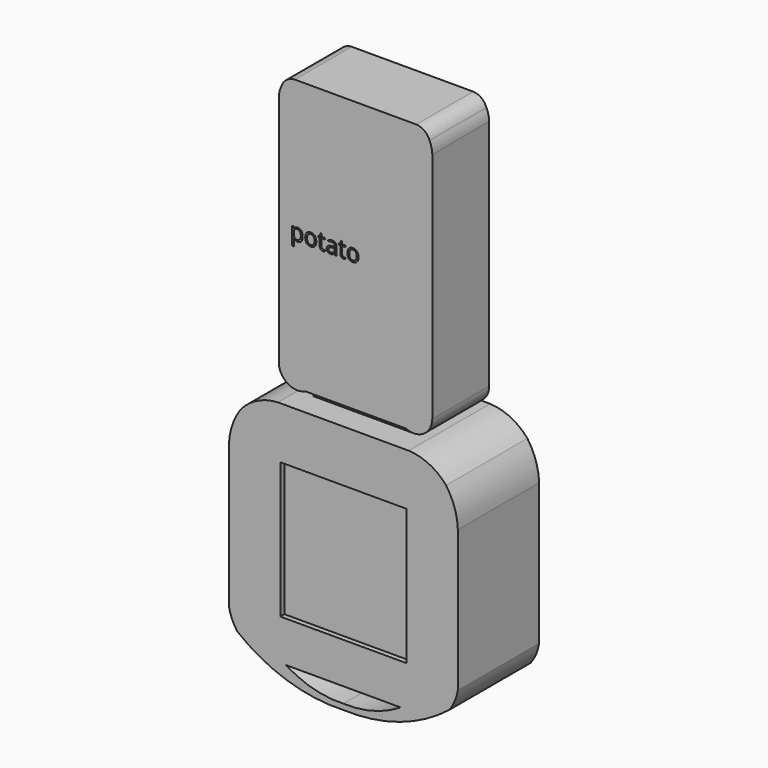
from build123d import *

# Parameters (mm, degrees)
F1_DEPTH      = 7
F1_DEPTH_BACK = 7
F0_W          = 19.7578053921
F0_H          = 1.6641734354
F2_DEPTH      = 5
F2_DEPTH_BACK = 5
F3_DEPTH      = 10
F3_DEPTH_BACK = 10
F0_W_2        = 24.8230153336
F0_H_2        = 26.7400959404
F0_R          = 11.1738098935
F4_DEPTH      = 9
F4_DEPTH_BACK = 8
F0_TEXT_SIZE  = 4.4513079855
F5_DEPTH      = 6
F5_DEPTH_BACK = 6
F6_DEPTH      = 10
F6_DEPTH_BACK = 8
F7_DEPTH      = 9
F7_DEPTH_BACK = 10


# Not quite as in the source:
# - Text() gives the source's letters only with a copy of the font that has no kerning and outlines rounded to 1/6400 em; it was checked with that copy


with BuildPart() as f1:
    # F0 (on Front) → F1 (new body, two sides)
    with BuildSketch(Plane.XZ) as f1_sk:
        with BuildLine():
            ThreePointArc((-0.3371863552, 48.0720782434), (-1.3488067521, 49.4383829581), (-2.9534097244, 50))
            Line((-2.9534097244, 50), (-3.174751997, 50))
            Line((-3.174751997, 50), (-14.9015085772, 50))
            Line((-14.9015085772, 50), (-26.6282651573, 50))
            Line((-26.6282651573, 50), (-26.8496074299, 50))
            ThreePointArc((-26.8496074299, 50), (-28.4542104022, 49.4383829581), (-29.4658307991, 48.0720782434))
            ThreePointArc((-29.4658307991, 48.0720782434), (-29.8531970792, 46.9903534646), (-30, 45.8507789675))
            Line((-30, 45.8507789675), (-30, 45.6348136067))
            Line((-30, 45.6348136067), (-30, 0))
            ThreePointArc((-30, 0), (-28.3036916744, -3.0972506092), (-24.7804112732, -3.3358265646))
            Line((-24.7804112732, -3.3358265646), (-5.0226058811, -3.3358265646))
            ThreePointArc((-5.0226058811, -3.3358265646), (-1.4993254799, -3.0972506092), (0.1969828457, 0))
            Line((0.1969828457, 0), (0.1969828457, 45.6348136067))
            Line((0.1969828457, 45.6348136067), (0.1969828457, 45.8507789675))
            ThreePointArc((0.1969828457, 45.8507789675), (0.0501799248, 46.9903534646), (-0.3371863552, 48.0720782434))
        make_face()
        with BuildLine():
            add(Edge.make_bspline(
                [(-25.5638879543, 22.3995790325), (-25.8257500569, 22.0744248945), (-26.2910508447, 22.0744248945)],
                knots=[0, 0, 0, 1, 1, 1], degree=2))
            add(Edge.make_bspline(
                [(-26.2910508447, 22.0744248945), (-26.5240489971, 22.0744248945), (-26.7163594124, 22.1603212283)],
                knots=[0, 0, 0, 1, 1, 1], degree=2))
            add(Edge.make_bspline(
                [(-26.7163594124, 22.1603212283), (-26.9086698277, 22.2462175621), (-27.0387314829, 22.4249653984)],
                knots=[0, 0, 0, 1, 1, 1], degree=2))
            Line((-27.0387314829, 22.4249653984), (-27.0651611241, 22.4249653984))
            add(Edge.make_bspline(
                [(-27.0651611241, 22.4249653984), (-27.0387314829, 22.2163103366), (-27.0387314829, 22.0292162978)],
                knots=[0, 0, 0, 1, 1, 1], degree=2))
            Line((-27.0387314829, 22.0292162978), (-27.0387314829, 21.0485375072))
            Line((-27.0387314829, 21.0485375072), (-27.3997047399, 21.0485375072))
            Line((-27.3997047399, 21.0485375072), (-27.3997047399, 24.5003877466))
            Line((-27.3997047399, 24.5003877466), (-27.1061966196, 24.5003877466))
            Line((-27.1061966196, 24.5003877466), (-27.0561194047, 24.1741903333))
            Line((-27.0561194047, 24.1741903333), (-27.0387314829, 24.1741903333))
            add(Edge.make_bspline(
                [(-27.0387314829, 24.1741903333), (-26.8996281084, 24.3703260914), (-26.7149683787, 24.4572657005)],
                knots=[0, 0, 0, 1, 1, 1], degree=2))
            add(Edge.make_bspline(
                [(-26.7149683787, 24.4572657005), (-26.5303086489, 24.5442053096), (-26.2910508447, 24.5442053096)],
                knots=[0, 0, 0, 1, 1, 1], degree=2))
            add(Edge.make_bspline(
                [(-26.2910508447, 24.5442053096), (-25.8174038544, 24.5442053096), (-25.559714853, 24.2200944469)],
                knots=[0, 0, 0, 1, 1, 1], degree=2))
            add(Edge.make_bspline(
                [(-25.559714853, 24.2200944469), (-25.3020258517, 23.8959835842), (-25.3020258517, 23.3117494111)],
                knots=[0, 0, 0, 1, 1, 1], degree=2))
            add(Edge.make_bspline(
                [(-25.3020258517, 23.3117494111), (-25.3020258517, 22.7247331705), (-25.5638879543, 22.3995790325)],
                knots=[0, 0, 0, 1, 1, 1], degree=2))
        make_face(mode=Mode.SUBTRACT)
        with BuildLine():
            add(Edge.make_bspline(
                [(-22.9104910848, 24.211400486), (-22.6159396892, 23.8785956624), (-22.6159396892, 23.3117494111)],
                knots=[0, 0, 0, 1, 1, 1], degree=2))
            add(Edge.make_bspline(
                [(-22.6159396892, 23.3117494111), (-22.6159396892, 22.7289062718), (-22.909100051, 22.4016655831)],
                knots=[0, 0, 0, 1, 1, 1], degree=2))
            add(Edge.make_bspline(
                [(-22.909100051, 22.4016655831), (-23.2022604129, 22.0744248945), (-23.7197249662, 22.0744248945)],
                knots=[0, 0, 0, 1, 1, 1], degree=2))
            add(Edge.make_bspline(
                [(-23.7197249662, 22.0744248945), (-24.0396627277, 22.0744248945), (-24.2872667344, 22.224656539)],
                knots=[0, 0, 0, 1, 1, 1], degree=2))
            add(Edge.make_bspline(
                [(-24.2872667344, 22.224656539), (-24.5348707411, 22.3748881835), (-24.6698010144, 22.6551814833)],
                knots=[0, 0, 0, 1, 1, 1], degree=2))
            add(Edge.make_bspline(
                [(-24.6698010144, 22.6551814833), (-24.8047312877, 22.935474783), (-24.8047312877, 23.3117494111)],
                knots=[0, 0, 0, 1, 1, 1], degree=2))
            add(Edge.make_bspline(
                [(-24.8047312877, 23.3117494111), (-24.8047312877, 23.8938970336), (-24.513309718, 24.2190511716)],
                knots=[0, 0, 0, 1, 1, 1], degree=2))
            add(Edge.make_bspline(
                [(-24.513309718, 24.2190511716), (-24.2218881483, 24.5442053096), (-23.704423595, 24.5442053096)],
                knots=[0, 0, 0, 1, 1, 1], degree=2))
            add(Edge.make_bspline(
                [(-23.704423595, 24.5442053096), (-23.2050424804, 24.5442053096), (-22.9104910848, 24.211400486)],
                knots=[0, 0, 0, 1, 1, 1], degree=2))
        make_face(mode=Mode.SUBTRACT)
        with BuildLine():
            add(Edge.make_bspline(
                [(-21.4940709735, 22.4879096754), (-21.3918299932, 22.3728016329), (-21.2137776737, 22.3728016329)],
                knots=[0, 0, 0, 1, 1, 1], degree=2))
            add(Edge.make_bspline(
                [(-21.2137776737, 22.3728016329), (-21.1177963453, 22.3728016329), (-21.0287701856, 22.3867119704)],
                knots=[0, 0, 0, 1, 1, 1], degree=2))
            add(Edge.make_bspline(
                [(-21.0287701856, 22.3867119704), (-20.9397440259, 22.4006223078), (-20.8875802604, 22.415923679)],
                knots=[0, 0, 0, 1, 1, 1], degree=2))
            Line((-20.8875802604, 22.415923679), (-20.8875802604, 22.1398034806))
            add(Edge.make_bspline(
                [(-20.8875802604, 22.1398034806), (-20.9460036777, 22.1119828057), (-21.0600684449, 22.0932038501)],
                knots=[0, 0, 0, 1, 1, 1], degree=2))
            add(Edge.make_bspline(
                [(-21.0600684449, 22.0932038501), (-21.174133212, 22.0744248945), (-21.2659414392, 22.0744248945)],
                knots=[0, 0, 0, 1, 1, 1], degree=2))
            add(Edge.make_bspline(
                [(-21.2659414392, 22.0744248945), (-21.9565896938, 22.0744248945), (-21.9565896938, 22.8026310603)],
                knots=[0, 0, 0, 1, 1, 1], degree=2))
            Line((-21.9565896938, 22.8026310603), (-21.9565896938, 24.2200944469))
            Line((-21.9565896938, 24.2200944469), (-22.2980884783, 24.2200944469))
            Line((-22.2980884783, 24.2200944469), (-22.2980884783, 24.3939736651))
            Line((-22.2980884783, 24.3939736651), (-21.9565896938, 24.5442053096))
            Line((-21.9565896938, 24.5442053096), (-21.8049670156, 25.0526281436))
            Line((-21.8049670156, 25.0526281436), (-21.5963119537, 25.0526281436))
            Line((-21.5963119537, 25.0526281436), (-21.5963119537, 24.5003877466))
            Line((-21.5963119537, 24.5003877466), (-20.9049681822, 24.5003877466))
            Line((-20.9049681822, 24.5003877466), (-20.9049681822, 24.2200944469))
            Line((-20.9049681822, 24.2200944469), (-21.5963119537, 24.2200944469))
            Line((-21.5963119537, 24.2200944469), (-21.5963119537, 22.8179324315))
            add(Edge.make_bspline(
                [(-21.5963119537, 22.8179324315), (-21.5963119537, 22.6030177178), (-21.4940709735, 22.4879096754)],
                knots=[0, 0, 0, 1, 1, 1], degree=2))
        make_face(mode=Mode.SUBTRACT)
        with BuildLine():
            Line((-18.6793141895, 22.1182424575), (-18.9470881855, 22.1182424575))
            Line((-18.9470881855, 22.1182424575), (-19.0187264234, 22.4576546914))
            Line((-19.0187264234, 22.4576546914), (-19.0361143452, 22.4576546914))
            add(Edge.make_bspline(
                [(-19.0361143452, 22.4576546914), (-19.2141666646, 22.2336982584), (-19.3911757087, 22.1540615765)],
                knots=[0, 0, 0, 1, 1, 1], degree=2))
            add(Edge.make_bspline(
                [(-19.3911757087, 22.1540615765), (-19.5681847528, 22.0744248945), (-19.8338721982, 22.0744248945)],
                knots=[0, 0, 0, 1, 1, 1], degree=2))
            add(Edge.make_bspline(
                [(-19.8338721982, 22.0744248945), (-20.1878902865, 22.0744248945), (-20.3888946627, 22.2573458321)],
                knots=[0, 0, 0, 1, 1, 1], degree=2))
            add(Edge.make_bspline(
                [(-20.3888946627, 22.2573458321), (-20.5898990389, 22.4402667696), (-20.5898990389, 22.776896936)],
                knots=[0, 0, 0, 1, 1, 1], degree=2))
            add(Edge.make_bspline(
                [(-20.5898990389, 22.776896936), (-20.5898990389, 23.498147933), (-19.436036547, 23.5329237767)],
                knots=[0, 0, 0, 1, 1, 1], degree=2))
            Line((-19.436036547, 23.5329237767), (-19.031941244, 23.5461385972))
            Line((-19.031941244, 23.5461385972), (-19.031941244, 23.6942836911))
            add(Edge.make_bspline(
                [(-19.031941244, 23.6942836911), (-19.031941244, 23.9745769908), (-19.1522656629, 24.1081162304)],
                knots=[0, 0, 0, 1, 1, 1], degree=2))
            add(Edge.make_bspline(
                [(-19.1522656629, 24.1081162304), (-19.2725900819, 24.24165547), (-19.5382775273, 24.24165547)],
                knots=[0, 0, 0, 1, 1, 1], degree=2))
            add(Edge.make_bspline(
                [(-19.5382775273, 24.24165547), (-19.8359587488, 24.24165547), (-20.2115378601, 24.0594300493)],
                knots=[0, 0, 0, 1, 1, 1], degree=2))
            Line((-20.2115378601, 24.0594300493), (-20.3228205598, 24.3355502478))
            add(Edge.make_bspline(
                [(-20.3228205598, 24.3355502478), (-20.146854791, 24.4308360594), (-19.9371564538, 24.4850863754)],
                knots=[0, 0, 0, 1, 1, 1], degree=2))
            add(Edge.make_bspline(
                [(-19.9371564538, 24.4850863754), (-19.7274581167, 24.5393366915), (-19.5160209874, 24.5393366915)],
                knots=[0, 0, 0, 1, 1, 1], degree=2))
            add(Edge.make_bspline(
                [(-19.5160209874, 24.5393366915), (-19.0903646613, 24.5393366915), (-18.8848394254, 24.3505038606)],
                knots=[0, 0, 0, 1, 1, 1], degree=2))
            add(Edge.make_bspline(
                [(-18.8848394254, 24.3505038606), (-18.6793141895, 24.1616710296), (-18.6793141895, 23.744360906)],
                knots=[0, 0, 0, 1, 1, 1], degree=2))
            Line((-18.6793141895, 23.744360906), (-18.6793141895, 22.1182424575))
        make_face(mode=Mode.SUBTRACT)
        with BuildLine():
            add(Edge.make_bspline(
                [(-17.4475538079, 22.4879096754), (-17.3453128276, 22.3728016329), (-17.1672605082, 22.3728016329)],
                knots=[0, 0, 0, 1, 1, 1], degree=2))
            add(Edge.make_bspline(
                [(-17.1672605082, 22.3728016329), (-17.0712791797, 22.3728016329), (-16.98225302, 22.3867119704)],
                knots=[0, 0, 0, 1, 1, 1], degree=2))
            add(Edge.make_bspline(
                [(-16.98225302, 22.3867119704), (-16.8932268603, 22.4006223078), (-16.8410630948, 22.415923679)],
                knots=[0, 0, 0, 1, 1, 1], degree=2))
            Line((-16.8410630948, 22.415923679), (-16.8410630948, 22.1398034806))
            add(Edge.make_bspline(
                [(-16.8410630948, 22.1398034806), (-16.8994865122, 22.1119828057), (-17.0135512793, 22.0932038501)],
                knots=[0, 0, 0, 1, 1, 1], degree=2))
            add(Edge.make_bspline(
                [(-17.0135512793, 22.0932038501), (-17.1276160464, 22.0744248945), (-17.2194242736, 22.0744248945)],
                knots=[0, 0, 0, 1, 1, 1], degree=2))
            add(Edge.make_bspline(
                [(-17.2194242736, 22.0744248945), (-17.9100725282, 22.0744248945), (-17.9100725282, 22.8026310603)],
                knots=[0, 0, 0, 1, 1, 1], degree=2))
            Line((-17.9100725282, 22.8026310603), (-17.9100725282, 24.2200944469))
            Line((-17.9100725282, 24.2200944469), (-18.2515713128, 24.2200944469))
            Line((-18.2515713128, 24.2200944469), (-18.2515713128, 24.3939736651))
            Line((-18.2515713128, 24.3939736651), (-17.9100725282, 24.5442053096))
            Line((-17.9100725282, 24.5442053096), (-17.75844985, 25.0526281436))
            Line((-17.75844985, 25.0526281436), (-17.5497947882, 25.0526281436))
            Line((-17.5497947882, 25.0526281436), (-17.5497947882, 24.5003877466))
            Line((-17.5497947882, 24.5003877466), (-16.8584510167, 24.5003877466))
            Line((-16.8584510167, 24.5003877466), (-16.8584510167, 24.2200944469))
            Line((-16.8584510167, 24.2200944469), (-17.5497947882, 24.2200944469))
            Line((-17.5497947882, 24.2200944469), (-17.5497947882, 22.8179324315))
            add(Edge.make_bspline(
                [(-17.5497947882, 22.8179324315), (-17.5497947882, 22.6030177178), (-17.4475538079, 22.4879096754)],
                knots=[0, 0, 0, 1, 1, 1], degree=2))
        make_face(mode=Mode.SUBTRACT)
        with BuildLine():
            add(Edge.make_bspline(
                [(-14.6039330737, 24.211400486), (-14.3093816781, 23.8785956624), (-14.3093816781, 23.3117494111)],
                knots=[0, 0, 0, 1, 1, 1], degree=2))
            add(Edge.make_bspline(
                [(-14.3093816781, 23.3117494111), (-14.3093816781, 22.7289062718), (-14.6025420399, 22.4016655831)],
                knots=[0, 0, 0, 1, 1, 1], degree=2))
            add(Edge.make_bspline(
                [(-14.6025420399, 22.4016655831), (-14.8957024018, 22.0744248945), (-15.4131669551, 22.0744248945)],
                knots=[0, 0, 0, 1, 1, 1], degree=2))
            add(Edge.make_bspline(
                [(-15.4131669551, 22.0744248945), (-15.7331047166, 22.0744248945), (-15.9807087233, 22.224656539)],
                knots=[0, 0, 0, 1, 1, 1], degree=2))
            add(Edge.make_bspline(
                [(-15.9807087233, 22.224656539), (-16.22831273, 22.3748881835), (-16.3632430033, 22.6551814833)],
                knots=[0, 0, 0, 1, 1, 1], degree=2))
            add(Edge.make_bspline(
                [(-16.3632430033, 22.6551814833), (-16.4981732766, 22.935474783), (-16.4981732766, 23.3117494111)],
                knots=[0, 0, 0, 1, 1, 1], degree=2))
            add(Edge.make_bspline(
                [(-16.4981732766, 23.3117494111), (-16.4981732766, 23.8938970336), (-16.2067517069, 24.2190511716)],
                knots=[0, 0, 0, 1, 1, 1], degree=2))
            add(Edge.make_bspline(
                [(-16.2067517069, 24.2190511716), (-15.9153301372, 24.5442053096), (-15.3978655839, 24.5442053096)],
                knots=[0, 0, 0, 1, 1, 1], degree=2))
            add(Edge.make_bspline(
                [(-15.3978655839, 24.5442053096), (-14.8984844693, 24.5442053096), (-14.6039330737, 24.211400486)],
                knots=[0, 0, 0, 1, 1, 1], degree=2))
        make_face(mode=Mode.SUBTRACT)
    extrude(amount=F1_DEPTH)
    extrude(f1_sk.sketch, amount=-F1_DEPTH_BACK)

    # F0 (on Front) → F2 (join, two sides)
    with BuildSketch(Plane.XZ) as f2_sk:
        with Locations((-14.9015085772, -4.1679132823)):
            Rectangle(F0_W, F0_H)
    extrude(amount=F2_DEPTH)
    extrude(f2_sk.sketch, amount=-F2_DEPTH_BACK)

    # F0 (on Front) → F3 (join, two sides)
    with BuildSketch(Plane.XZ) as f3_sk:
        with BuildLine():
            Line((-4.7804112732, -5), (-5.0226058811, -5))
            Line((-5.0226058811, -5), (-24.7804112732, -5))
            Line((-24.7804112732, -5), (-26.8505178392, -5))
            Line((-26.8505178392, -5), (-27.7755146487, -5))
            ThreePointArc((-27.7755146487, -5), (-31.8249756764, -6.0389542539), (-35.1200683324, -8.6118757345))
            ThreePointArc((-35.1200683324, -8.6118757345), (-36.7849914207, -11.9049706979), (-37.4285317957, -15.5384675143))
            Line((-37.4285317957, -15.5384675143), (-37.4285317957, -43.3827936649))
            ThreePointArc((-37.4285317957, -43.3827936649), (-36.8364830132, -45.4381899261), (-35.7731175765, -47.2941073539))
            ThreePointArc((-35.7731175765, -47.2941073539), (-25.9517344842, -52.5831834244), (-14.9015085772, -54.1084371507))
            ThreePointArc((-14.9015085772, -54.1084371507), (-3.8512826702, -52.5831834244), (5.9701004222, -47.2941073539))
            ThreePointArc((5.9701004222, -47.2941073539), (7.0334658589, -45.4381899261), (7.6255146414, -43.3827936649))
            Line((7.6255146414, -43.3827936649), (7.6255146414, -15.5384675143))
            ThreePointArc((7.6255146414, -15.5384675143), (6.9819742664, -11.9049706979), (5.317051178, -8.6118757345))
            ThreePointArc((5.317051178, -8.6118757345), (2.0219585221, -6.0389542539), (-2.0275025056, -5))
            Line((-2.0275025056, -5), (-2.9524993151, -5))
            Line((-2.9524993151, -5), (-4.7804112732, -5))
        make_face()
        with BuildLine():
            ThreePointArc((-3.6269985139, -50), (-9.0351634562, -52.3629954978), (-14.9015085772, -53.0095174909))
            ThreePointArc((-14.9015085772, -53.0095174909), (-20.7678536981, -52.3629954978), (-26.1760186404, -50))
            Line((-26.1760186404, -50), (-3.6269985139, -50))
        make_face(mode=Mode.SUBTRACT)
        Polygon((-2.4900009104, -41.9538753285), (-27.313016244, -41.9538753285), (-28.6317821592, -41.9538753285), (-28.6317821592, -13.223904185), (-1.1990642376, -13.223904185), (-1.1990642376, -41.9538753285), align=None, mode=Mode.SUBTRACT)
    extrude(amount=F3_DEPTH)
    extrude(f3_sk.sketch, amount=-F3_DEPTH_BACK)

    # F0 (on Front) → F4 (join, two sides)
    with BuildSketch(Plane.XZ) as f4_sk:
        with Locations((-14.9015085772, -28.5838273583)):
            Rectangle(F0_W_2, F0_H_2)
        with Locations((-14.8883853108, -28.2334722579)):
            Circle(F0_R, mode=Mode.SUBTRACT)
    extrude(amount=F4_DEPTH)
    extrude(f4_sk.sketch, amount=-F4_DEPTH_BACK)

    # F0 (on Front) → F6 (join, two sides)
    with BuildSketch(Plane.XZ) as f6_sk:
        Polygon((-27.313016244, -41.9538753285), (-27.313016244, -15.2137793881), (-2.4900009104, -15.2137793881), (-2.4900009104, -41.9538753285), (-1.1990642376, -41.9538753285), (-1.1990642376, -13.223904185), (-28.6317821592, -13.223904185), (-28.6317821592, -41.9538753285), align=None)
    extrude(amount=F6_DEPTH)
    extrude(f6_sk.sketch, amount=-F6_DEPTH_BACK)

    # F0 (on Front) → F7 (join, two sides)
    with BuildSketch(Plane.XZ) as f7_sk:
        with Locations((-14.8883853108, -28.2334722579)):
            Circle(F0_R)
    extrude(amount=F7_DEPTH)
    extrude(f7_sk.sketch, amount=-F7_DEPTH_BACK)


with BuildPart() as f1b:
    # F0 (on Front) → F1, piece 2 (new body, two sides)
    with BuildSketch(Plane.XZ) as f1_2_sk:
        with BuildLine():
            add(Edge.make_bspline(
                [(-24.2500565817, 24.0048319748), (-24.4305432102, 23.7721815809), (-24.4305432102, 23.3117494111)],
                knots=[0, 0, 0, 1, 1, 1], degree=2))
            add(Edge.make_bspline(
                [(-24.4305432102, 23.3117494111), (-24.4305432102, 22.8547948257), (-24.2479700311, 22.61588478)],
                knots=[0, 0, 0, 1, 1, 1], degree=2))
            add(Edge.make_bspline(
                [(-24.2479700311, 22.61588478), (-24.065396852, 22.3769747342), (-23.7113787637, 22.3769747342)],
                knots=[0, 0, 0, 1, 1, 1], degree=2))
            add(Edge.make_bspline(
                [(-23.7113787637, 22.3769747342), (-23.3566651586, 22.3769747342), (-23.1730487042, 22.6148415046)],
                knots=[0, 0, 0, 1, 1, 1], degree=2))
            add(Edge.make_bspline(
                [(-23.1730487042, 22.6148415046), (-22.9894322498, 22.8527082751), (-22.9894322498, 23.3117494111)],
                knots=[0, 0, 0, 1, 1, 1], degree=2))
            add(Edge.make_bspline(
                [(-22.9894322498, 23.3117494111), (-22.9894322498, 23.765921929), (-23.1730487042, 24.0017021489)],
                knots=[0, 0, 0, 1, 1, 1], degree=2))
            add(Edge.make_bspline(
                [(-23.1730487042, 24.0017021489), (-23.3566651586, 24.2374823687), (-23.715551865, 24.2374823687)],
                knots=[0, 0, 0, 1, 1, 1], degree=2))
            add(Edge.make_bspline(
                [(-23.715551865, 24.2374823687), (-24.0695699532, 24.2374823687), (-24.2500565817, 24.0048319748)],
                knots=[0, 0, 0, 1, 1, 1], degree=2))
        make_face()
    extrude(amount=F1_DEPTH)
    extrude(f1_2_sk.sketch, amount=-F1_DEPTH_BACK)


with BuildPart() as f1c:
    # F0 (on Front) → F1, piece 3 (new body, two sides)
    with BuildSketch(Plane.XZ) as f1_3_sk:
        with BuildLine():
            add(Edge.make_bspline(
                [(-25.8511364227, 23.9996155983), (-26.0260589162, 24.2374823687), (-26.3432146102, 24.2374823687)],
                knots=[0, 0, 0, 1, 1, 1], degree=2))
            add(Edge.make_bspline(
                [(-26.3432146102, 24.2374823687), (-26.7083609684, 24.2374823687), (-26.871459675, 24.0354347172)],
                knots=[0, 0, 0, 1, 1, 1], degree=2))
            add(Edge.make_bspline(
                [(-26.871459675, 24.0354347172), (-27.0345583817, 23.8333870657), (-27.0387314829, 23.3917338515)],
                knots=[0, 0, 0, 1, 1, 1], degree=2))
            Line((-27.0387314829, 23.3917338515), (-27.0387314829, 23.3117494111))
            add(Edge.make_bspline(
                [(-27.0387314829, 23.3117494111), (-27.0387314829, 22.809586229), (-26.871459675, 22.5932804816)],
                knots=[0, 0, 0, 1, 1, 1], degree=2))
            add(Edge.make_bspline(
                [(-26.871459675, 22.5932804816), (-26.7041878671, 22.3769747342), (-26.3348684077, 22.3769747342)],
                knots=[0, 0, 0, 1, 1, 1], degree=2))
            add(Edge.make_bspline(
                [(-26.3348684077, 22.3769747342), (-26.0260589162, 22.3769747342), (-25.8511364227, 22.6270130499)],
                knots=[0, 0, 0, 1, 1, 1], degree=2))
            add(Edge.make_bspline(
                [(-25.8511364227, 22.6270130499), (-25.6762139292, 22.8770513657), (-25.6762139292, 23.3159225124)],
                knots=[0, 0, 0, 1, 1, 1], degree=2))
            add(Edge.make_bspline(
                [(-25.6762139292, 23.3159225124), (-25.6762139292, 23.7617488278), (-25.8511364227, 23.9996155983)],
                knots=[0, 0, 0, 1, 1, 1], degree=2))
        make_face()
    extrude(amount=F1_DEPTH)
    extrude(f1_3_sk.sketch, amount=-F1_DEPTH_BACK)


with BuildPart() as f1d:
    # F0 (on Front) → F1, piece 4 (new body, two sides)
    with BuildSketch(Plane.XZ) as f1_4_sk:
        with BuildLine():
            add(Edge.make_bspline(
                [(-20.0932999918, 22.4746948548), (-19.9750621234, 22.3728016329), (-19.7622339603, 22.3728016329)],
                knots=[0, 0, 0, 1, 1, 1], degree=2))
            add(Edge.make_bspline(
                [(-19.7622339603, 22.3728016329), (-19.4249082771, 22.3728016329), (-19.2325978617, 22.5574613626)],
                knots=[0, 0, 0, 1, 1, 1], degree=2))
            add(Edge.make_bspline(
                [(-19.2325978617, 22.5574613626), (-19.0402874464, 22.7421210924), (-19.0402874464, 23.0745781575)],
                knots=[0, 0, 0, 1, 1, 1], degree=2))
            Line((-19.0402874464, 23.0745781575), (-19.0402874464, 23.2894928712))
            Line((-19.0402874464, 23.2894928712), (-19.4012607034, 23.2748870169))
            add(Edge.make_bspline(
                [(-19.4012607034, 23.2748870169), (-19.8317856476, 23.2595856457), (-20.0216617539, 23.1410000189)],
                knots=[0, 0, 0, 1, 1, 1], degree=2))
            add(Edge.make_bspline(
                [(-20.0216617539, 23.1410000189), (-20.2115378601, 23.0224143921), (-20.2115378601, 22.7727238348)],
                knots=[0, 0, 0, 1, 1, 1], degree=2))
            add(Edge.make_bspline(
                [(-20.2115378601, 22.7727238348), (-20.2115378601, 22.5765880766), (-20.0932999918, 22.4746948548)],
                knots=[0, 0, 0, 1, 1, 1], degree=2))
        make_face()
    extrude(amount=F1_DEPTH)
    extrude(f1_4_sk.sketch, amount=-F1_DEPTH_BACK)


with BuildPart() as f1e:
    # F0 (on Front) → F1, piece 5 (new body, two sides)
    with BuildSketch(Plane.XZ) as f1_5_sk:
        with BuildLine():
            add(Edge.make_bspline(
                [(-15.9434985706, 24.0048319748), (-16.1239851991, 23.7721815809), (-16.1239851991, 23.3117494111)],
                knots=[0, 0, 0, 1, 1, 1], degree=2))
            add(Edge.make_bspline(
                [(-16.1239851991, 23.3117494111), (-16.1239851991, 22.8547948257), (-15.94141202, 22.61588478)],
                knots=[0, 0, 0, 1, 1, 1], degree=2))
            add(Edge.make_bspline(
                [(-15.94141202, 22.61588478), (-15.7588388409, 22.3769747342), (-15.4048207526, 22.3769747342)],
                knots=[0, 0, 0, 1, 1, 1], degree=2))
            add(Edge.make_bspline(
                [(-15.4048207526, 22.3769747342), (-15.0501071475, 22.3769747342), (-14.8664906931, 22.6148415046)],
                knots=[0, 0, 0, 1, 1, 1], degree=2))
            add(Edge.make_bspline(
                [(-14.8664906931, 22.6148415046), (-14.6828742387, 22.8527082751), (-14.6828742387, 23.3117494111)],
                knots=[0, 0, 0, 1, 1, 1], degree=2))
            add(Edge.make_bspline(
                [(-14.6828742387, 23.3117494111), (-14.6828742387, 23.765921929), (-14.8664906931, 24.0017021489)],
                knots=[0, 0, 0, 1, 1, 1], degree=2))
            add(Edge.make_bspline(
                [(-14.8664906931, 24.0017021489), (-15.0501071475, 24.2374823687), (-15.4089938539, 24.2374823687)],
                knots=[0, 0, 0, 1, 1, 1], degree=2))
            add(Edge.make_bspline(
                [(-15.4089938539, 24.2374823687), (-15.7630119421, 24.2374823687), (-15.9434985706, 24.0048319748)],
                knots=[0, 0, 0, 1, 1, 1], degree=2))
        make_face()
    extrude(amount=F1_DEPTH)
    extrude(f1_5_sk.sketch, amount=-F1_DEPTH_BACK)


with BuildPart() as f5:
    # F0 (on Front) → F5 (new body, two sides)
    with BuildSketch(Plane.XZ) as f5_sk:
        with Locations((-27.7822390199, 22.1182424575)):
            Text('potato', F0_TEXT_SIZE, font='Open Sans', text_align=(TextAlign.LEFT, TextAlign.BOTTOM))
    extrude(amount=F5_DEPTH)
    extrude(f5_sk.sketch, amount=-F5_DEPTH_BACK)


solid = Compound([f1.part, f1b.part, f1c.part, f1d.part, f1e.part, f5.part])
